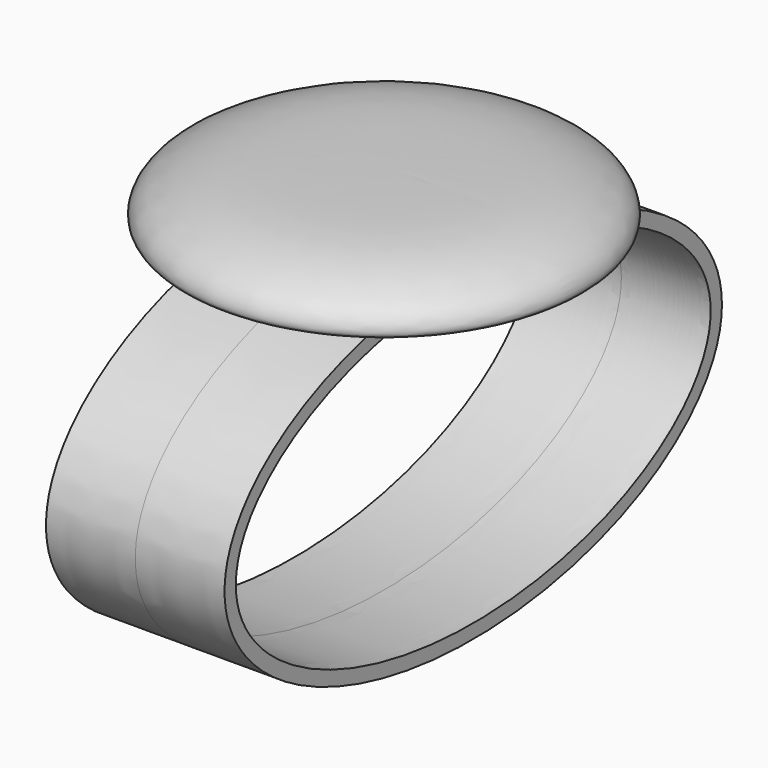
from build123d import *

# Parameters (mm, degrees)
F3_DEPTH = 28.956


# Not quite as in the source:
# - the dataset's text gives a spline's control points without its knots; the knots are read off the source's solid


with BuildPart() as f1:
    # F0 (on Front) → F1 (revolve)
    with BuildSketch(Plane.XZ):
        with BuildLine():
            add(Edge.make_bspline(
                [(0, 16.4452996105), (30.8186020702, 16.4452996105), (43.983156173, 15.5098561698), (57.6907424529, 10.878360347), (65.0685794541, 5.9684141276), (65.29904237, 0), (61.642778678, 0)],
                knots=[0, 0, 0, 0, 0.4462200986, 0.6598383382, 0.850023127, 1, 1, 1, 1], degree=3))
            Line((0, 16.4452996105), (0, 0))
            Line((0, 0), (61.642778678, 0))
        make_face()
    revolve(axis=Axis((0, 0, 8.2226498052), (0, 0, -1)))


with BuildPart() as f3:
    # F2 (on Right) → F3 (new body, symmetric)
    with BuildSketch(Plane.YZ):
        with BuildLine():
            add(Edge.make_bspline(
                [(0, -0.2640799607), (-174.5732618017, -0.2640799607), (-87.2866309008, -82.1807022678), (0, -164.097324575), (87.2866309008, -82.1807022678), (174.5732618017, -0.2640799607), (0, -0.2640799607)],
                knots=[4.7123889804, 4.7123889804, 4.7123889804, 6.8067840828, 6.8067840828, 8.9011791852, 8.9011791852, 10.9955742876, 10.9955742876, 10.9955742876], degree=2, weights=[1, 0.5, 1, 0.5, 1, 0.5, 1]))
        make_face()
        with BuildLine():
            add(Edge.make_bspline(
                [(-96.2179228663, -54.8751614988), (-96.2179228663, -55.6395041682), (-96.1478272303, -57.1681895069), (-95.7297661828, -60.2097462459), (-94.6868854018, -63.9995987995), (-92.5895614096, -68.5281474967), (-89.6299993115, -73.0121100269), (-85.8024153279, -77.4063276161), (-81.8948466173, -80.9493546032), (-78.3465315575, -83.6855517255), (-75.4765641489, -85.6823056635), (-72.4024200782, -87.6164613491), (-69.1213783583, -89.4851012114), (-65.6590299931, -91.270236762), (-62.0460611674, -92.9564523887), (-58.2851114425, -94.5437945315), (-53.0868648896, -96.5232992594), (-46.2654981106, -98.7342960844), (-37.6323125055, -100.9449978286), (-28.6213226262, -102.6942415931), (-20.855389462, -103.7526777965), (-14.5232272738, -104.3516025507), (-9.7231461471, -104.6749107046), (-5.687470505, -104.8378147204), (-2.4426409998, -104.9032837925), (0, -104.9197274169), (2.4426409998, -104.9032837925), (5.687470505, -104.8378147204), (9.7231461471, -104.6749107046), (14.5232272738, -104.3516025507), (20.855389462, -103.7526777965), (28.6213226262, -102.6942415931), (37.6323125055, -100.9449978286), (46.2654981106, -98.7342960844), (53.0868648896, -96.5232992594), (58.2851114425, -94.5437945315), (62.0460611674, -92.9564523887), (65.6590299931, -91.270236762), (69.1213783583, -89.4851012114), (72.4024200782, -87.6164613491), (75.4765641489, -85.6823056635), (78.3465315575, -83.6855517255), (81.8948466173, -80.9493546032), (85.8024153279, -77.4063276161), (89.6299993115, -73.0121100269), (92.5895614096, -68.5281474967), (94.6868854018, -63.9995987995), (95.7297661828, -60.2097462459), (96.1478272303, -57.1681895069), (96.2529706844, -54.8751614988), (96.1478272303, -52.5821334907), (95.7297661828, -49.5405767517), (94.6868854018, -45.7507241981), (92.5895614096, -41.2221755008), (89.6299993115, -36.7382129707), (85.8024153279, -32.3439953814), (81.8948466173, -28.8009683943), (78.3465315575, -26.0647712721), (75.4765641489, -24.0680173341), (72.4024200782, -22.1338616485), (69.1213783583, -20.2652217862), (65.6590299931, -18.4800862356), (62.0460611674, -16.7938706089), (58.2851114425, -15.2065284661), (53.0868648896, -13.2270237381), (46.2654981106, -11.0160269132), (37.6323125055, -8.805325169), (28.6213226262, -7.0560814045), (20.855389462, -5.997645201), (14.5232272738, -5.3987204469), (9.7231461471, -5.0754122929), (5.687470505, -4.9125082771), (2.4426409998, -4.847039205), (0, -4.8305955807), (-2.4426409998, -4.847039205), (-5.687470505, -4.9125082771), (-9.7231461471, -5.0754122929), (-14.5232272738, -5.3987204469), (-20.855389462, -5.997645201), (-28.6213226262, -7.0560814045), (-37.6323125055, -8.805325169), (-46.2654981106, -11.0160269132), (-53.0868648896, -13.2270237381), (-58.2851114425, -15.2065284661), (-62.0460611674, -16.7938706089), (-65.6590299931, -18.4800862356), (-69.1213783583, -20.2652217862), (-72.4024200782, -22.1338616485), (-75.4765641489, -24.0680173341), (-78.3465315575, -26.0647712721), (-81.8948466173, -28.8009683943), (-85.8024153279, -32.3439953814), (-89.6299993115, -36.7382129707), (-92.5895614096, -41.2221755008), (-94.6868854018, -45.7507241981), (-95.7297661828, -49.5405767517), (-96.1478272303, -52.5821334907), (-96.2179228663, -54.1108188294), (-96.2179228663, -54.8751614988)],
                knots=[0, 0, 0, 0, 0.0078125, 0.015625, 0.03125, 0.046875, 0.0625, 0.078125, 0.09375, 0.1015625, 0.109375, 0.1171875, 0.125, 0.1328125, 0.140625, 0.1484375, 0.15625, 0.171875, 0.1875, 0.203125, 0.21875, 0.2265625, 0.234375, 0.2421875, 0.24609375, 0.25, 0.25390625, 0.2578125, 0.265625, 0.2734375, 0.28125, 0.296875, 0.3125, 0.328125, 0.34375, 0.3515625, 0.359375, 0.3671875, 0.375, 0.3828125, 0.390625, 0.3984375, 0.40625, 0.421875, 0.4375, 0.453125, 0.46875, 0.484375, 0.4921875, 0.5, 0.5078125, 0.515625, 0.53125, 0.546875, 0.5625, 0.578125, 0.59375, 0.6015625, 0.609375, 0.6171875, 0.625, 0.6328125, 0.640625, 0.6484375, 0.65625, 0.671875, 0.6875, 0.703125, 0.71875, 0.7265625, 0.734375, 0.7421875, 0.74609375, 0.75, 0.75390625, 0.7578125, 0.765625, 0.7734375, 0.78125, 0.796875, 0.8125, 0.828125, 0.84375, 0.8515625, 0.859375, 0.8671875, 0.875, 0.8828125, 0.890625, 0.8984375, 0.90625, 0.921875, 0.9375, 0.953125, 0.96875, 0.984375, 0.9921875, 1, 1, 1, 1], degree=3))
        make_face(mode=Mode.SUBTRACT)
    extrude(amount=F3_DEPTH, both=True)


solid = Compound([f1.part, f3.part])
